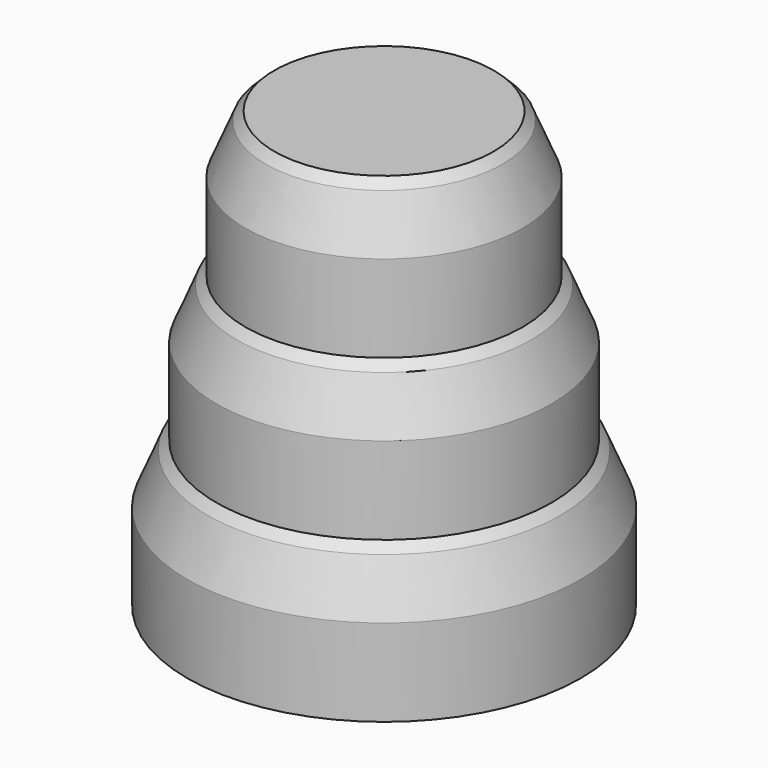
from build123d import *

# Parameters (mm, degrees)
F0_R     = 34.44374921
F1_DEPTH = 25.4
F2_SIZE  = 5.08
F3_SIZE  = 5.08
F4_DEPTH = 25.4
F5_SIZE  = 5.08
F6_DEPTH = 25.4
F7_SIZE  = 5.08
F8_SIZE  = 5.08


# Not quite as in the source:
# - two fillets or chamfers of one size are made in one step


with BuildPart() as f1:
    # F0 (on Top) → F1 (new body)
    with BuildSketch(Plane.XY):
        with Locations((-39.9288013577, 17.5260007381)):
            Circle(F0_R)
    extrude(amount=F1_DEPTH)

    # F2
    f2_edges = [f1.edges().sort_by_distance(p)[0] for p in [
        (-74.372551, 17.526001, 25.4),
    ]]
    chamfer(f2_edges, length=F2_SIZE)

    # F3
    f3_edges = [f1.edges().sort_by_distance(p)[0] for p in [
        (-74.372551, 17.526001, 20.32),
    ]]
    chamfer(f3_edges, length=F3_SIZE)

    # F4 (add): a face of the model
    f4_faces = [f1.faces().sort_by_distance(p)[0] for p in [
        (-39.9288013577, 17.5260007381, 25.4),
    ]]
    extrude(f4_faces, amount=F4_DEPTH)

    # F5
    f5_edges = [f1.edges().sort_by_distance(p)[0] for p in [
        (-69.292551, 17.526001, 50.8),
    ]]
    chamfer(f5_edges, length=F5_SIZE)

    # F6 (add): a face of the model
    f6_faces = [f1.faces().sort_by_distance(p)[0] for p in [
        (-39.9288013577, 17.5260007381, 50.8),
    ]]
    extrude(f6_faces, amount=F6_DEPTH)

    # F7
    f7_edges = [f1.edges().sort_by_distance(p)[0] for p in [
        (-69.292551, 17.526001, 45.72),
        (-64.212551, 17.526001, 76.2),
    ]]
    chamfer(f7_edges, length=F7_SIZE)

    # F8
    f8_edges = [f1.edges().sort_by_distance(p)[0] for p in [
        (-64.212551, 17.526001, 71.12),
    ]]
    chamfer(f8_edges, length=F8_SIZE)


solid = f1.part
